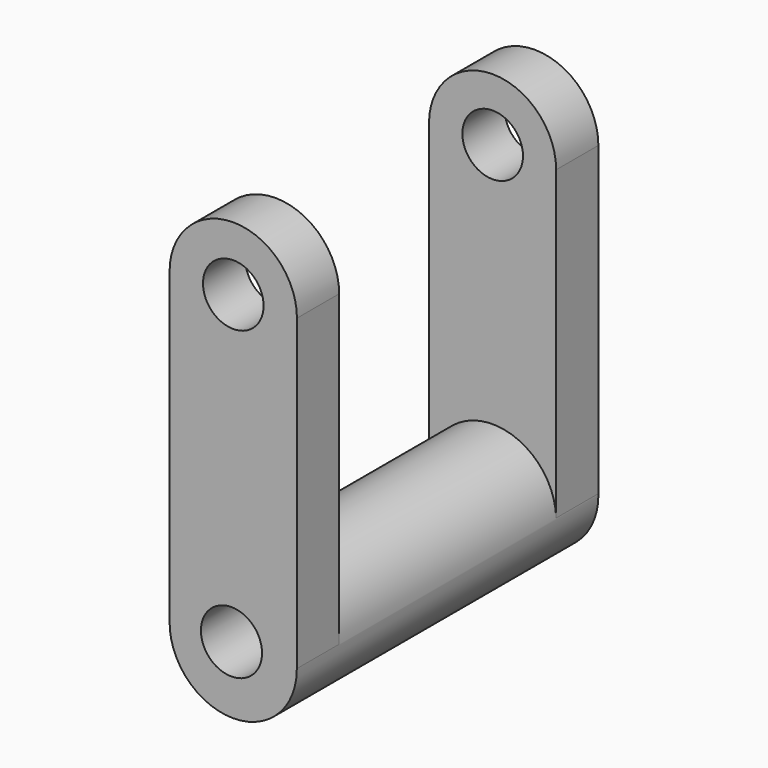
from build123d import *

# Parameters (mm, degrees)
F0_R      = 21.4164389033
F1_DEPTH  = 127
F2_W      = 42.8202235004
F2_H      = 103.2743248374
F3_DEPTH  = 17.78
F5_DEPTH  = 17.78
F6_R      = 7.3683109371
F7_DEPTH  = 273
F8_R      = 10.2975296605
F9_DEPTH  = 127.001
F11_DEPTH = 17.78
F13_DEPTH = 17.78
F14_R     = 10.2092328794
F15_DEPTH = 127.001


# Not quite as in the source:
# - an extrude ends at something that could not be found from the text; its depth is read off the source's solid


with BuildPart() as f1:
    # F0 (on Front) → F1 (new body)
    with BuildSketch(Plane.XZ):
        with Locations((25.1603480428, 31.716234982)):
            Circle(F0_R)
    extrude(amount=F1_DEPTH)

    # F2 (on face) → F3 (join)
    with BuildSketch(Plane(origin=(0, 0, 0), x_dir=(-1, 0, 0), z_dir=(0, 1, 0))):
        with Locations((-25.1603480428, 83.8739453241)):
            Rectangle(F2_W, F2_H)
    extrude(amount=-F3_DEPTH)

    # F4 (on face) → F5 (join)
    with BuildSketch(Plane.XZ.offset(127)):
        Polygon((3.7453082572, 31.961033423), (46.5753878285, 31.961033423), (46.636801213, 135.9289437532), (3.7453082572, 135.9289437532), align=None)
    extrude(amount=-F5_DEPTH)

    # F6 (on Front) → F7 (cut, through all)
    with BuildSketch(Plane.XZ):
        with Locations((25.2368301153, 31.4926542342)):
            Circle(F6_R)
    extrude(amount=-F7_DEPTH, mode=Mode.SUBTRACT)

    # F8 (on Front) → F9 (cut, through all)
    with BuildSketch(Plane.XZ):
        with Locations((24.5855599642, 32.795201987)):
            Circle(F8_R)
    extrude(amount=F9_DEPTH, mode=Mode.SUBTRACT)

    # F10 (on face) → F11 (join)
    with BuildSketch(Plane.XZ.offset(127)):
        with BuildLine():
            Line((3.7453082572, 135.9289437532), (46.636801213, 135.9289437532))
            ThreePointArc((46.636801213, 135.9289437532), (25.1910547351, 157.3873618801), (3.7453082572, 135.9289437532))
        make_face()
    extrude(amount=-F11_DEPTH)

    # F12 (on face) → F13 (join)
    with BuildSketch(Plane(origin=(0, 0, 0), x_dir=(-1, 0, 0), z_dir=(0, 1, 0))):
        with BuildLine():
            Line((-46.5704597931, 135.5111077428), (-3.7502362926, 135.5111077428))
            ThreePointArc((-3.7502362926, 135.5111077428), (-25.1603480428, 156.921219493), (-46.5704597931, 135.5111077428))
        make_face()
    extrude(amount=-F13_DEPTH)

    # F14 (on face) → F15 (cut, through all)
    with BuildSketch(Plane.XZ.offset(127)):
        with Locations((25.1910547351, 135.9416116608)):
            Circle(F14_R)
    extrude(amount=-F15_DEPTH, mode=Mode.SUBTRACT)


solid = f1.part
